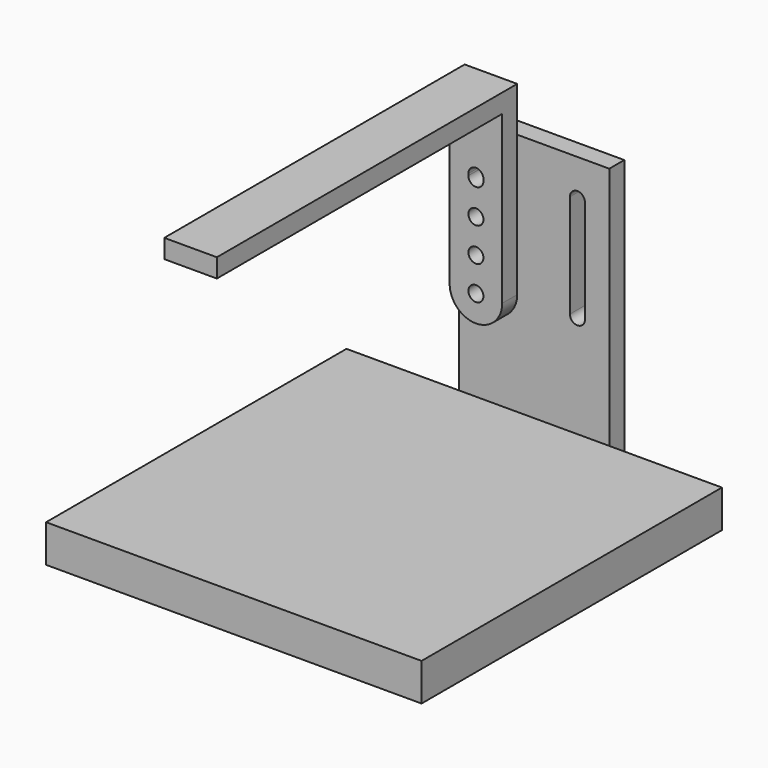
from build123d import *

# Parameters (mm, degrees)
F3_W      = 100
F3_H      = 100
F4_DEPTH  = 10
F5_W      = 40
F5_H      = 65
F5_H_2    = 10
F6_DEPTH  = 5
F7_W      = 14
F7_H      = 6.915564537
F7_H_2    = 5
F8_DEPTH  = 5
F9_W      = 14
F9_H      = 95
F10_DEPTH = 5


with BuildPart() as f4:
    # F3 (on Top) → F4 (new body)
    with BuildSketch(Plane.XY):
        Rectangle(F3_W, F3_H)
    extrude(amount=F4_DEPTH)

    # F5 (on face) → F6 (join)
    with BuildSketch(Plane(origin=(0, 50, 0), x_dir=(-1, 0, 0), z_dir=(0, 1, 0))):
        with Locations((0, 42.5)):
            Rectangle(F5_W, F5_H)
        with BuildLine():
            Line((-13.518457301, 37.5), (-13.518457301, 65))
            ThreePointArc((-13.518457301, 65), (-11.518457301, 67), (-9.518457301, 65))
            Line((-9.518457301, 65), (-9.518457301, 37.5))
            ThreePointArc((-9.518457301, 37.5), (-11.518457301, 35.5), (-13.518457301, 37.5))
        make_face(mode=Mode.SUBTRACT)
        with BuildLine():
            Line((9.518457301, 37.5), (9.518457301, 65))
            ThreePointArc((9.518457301, 65), (11.518457301, 67), (13.518457301, 65))
            Line((13.518457301, 65), (13.518457301, 37.5))
            ThreePointArc((13.518457301, 37.5), (11.518457301, 35.5), (9.518457301, 37.5))
        make_face(mode=Mode.SUBTRACT)
        with Locations((0, 5)):
            Rectangle(F5_W, F5_H_2)
    extrude(amount=F6_DEPTH)


with BuildPart() as f8:
    # F7 (on face) → F8 (new body)
    with BuildSketch(Plane(origin=(0, 50, 0), x_dir=(-1, 0, 0), z_dir=(0, 1, 0))):
        with BuildLine():
            Line((4.518457301, 75), (4.518457301, 37.5))
            ThreePointArc((4.518457301, 37.5), (11.518457301, 30.5), (18.518457301, 37.5))
            Line((18.518457301, 37.5), (18.518457301, 75))
            Line((18.518457301, 75), (4.518457301, 75))
        make_face()
        with BuildLine():
            Line((13.518457301, 46.5), (13.518457301, 37.5))
            ThreePointArc((13.518457301, 37.5), (11.518457301, 35.5), (9.518457301, 37.5))
            Line((9.518457301, 37.5), (9.518457301, 46.5))
            Line((9.518457301, 46.5), (9.518457301, 55.5))
            Line((9.518457301, 55.5), (9.518457301, 64.5))
            Line((9.518457301, 64.5), (9.518457301, 65))
            ThreePointArc((9.518457301, 65), (11.518457301, 67), (13.518457301, 65))
            Line((13.518457301, 65), (13.518457301, 64.5))
            Line((13.518457301, 64.5), (13.518457301, 55.5))
            Line((13.518457301, 55.5), (13.518457301, 46.5))
        make_face(mode=Mode.SUBTRACT)
        with Locations((11.518457301, 78.4577822685)):
            Rectangle(F7_W, F7_H)
        with Locations((11.518457301, 84.415564537)):
            Rectangle(F7_W, F7_H_2)
        with BuildLine():
            ThreePointArc((9.518457301, 37.5), (11.518457301, 39.5), (13.518457301, 37.5))
            Line((13.518457301, 37.5), (13.518457301, 46.5))
            ThreePointArc((13.518457301, 46.5), (11.518457301, 44.5), (9.518457301, 46.5))
            Line((9.518457301, 46.5), (9.518457301, 37.5))
        make_face()
        with BuildLine():
            ThreePointArc((9.518457301, 46.5), (11.518457301, 48.5), (13.518457301, 46.5))
            Line((13.518457301, 46.5), (13.518457301, 55.5))
            ThreePointArc((13.518457301, 55.5), (11.518457301, 53.5), (9.518457301, 55.5))
            Line((9.518457301, 55.5), (9.518457301, 46.5))
        make_face()
        with BuildLine():
            ThreePointArc((9.518457301, 55.5), (11.518457301, 57.5), (13.518457301, 55.5))
            Line((13.518457301, 55.5), (13.518457301, 64.5))
            ThreePointArc((13.518457301, 64.5), (11.518457301, 62.5), (9.518457301, 64.5))
            Line((9.518457301, 64.5), (9.518457301, 55.5))
        make_face()
    extrude(amount=-F8_DEPTH)

    # F9 (on face) → F10 (join)
    with BuildSketch(Plane.XY.offset(86.915564537)):
        with Locations((-11.518457301, -2.5)):
            Rectangle(F9_W, F9_H)
    extrude(amount=-F10_DEPTH)


solid = Compound([f4.part, f8.part])
